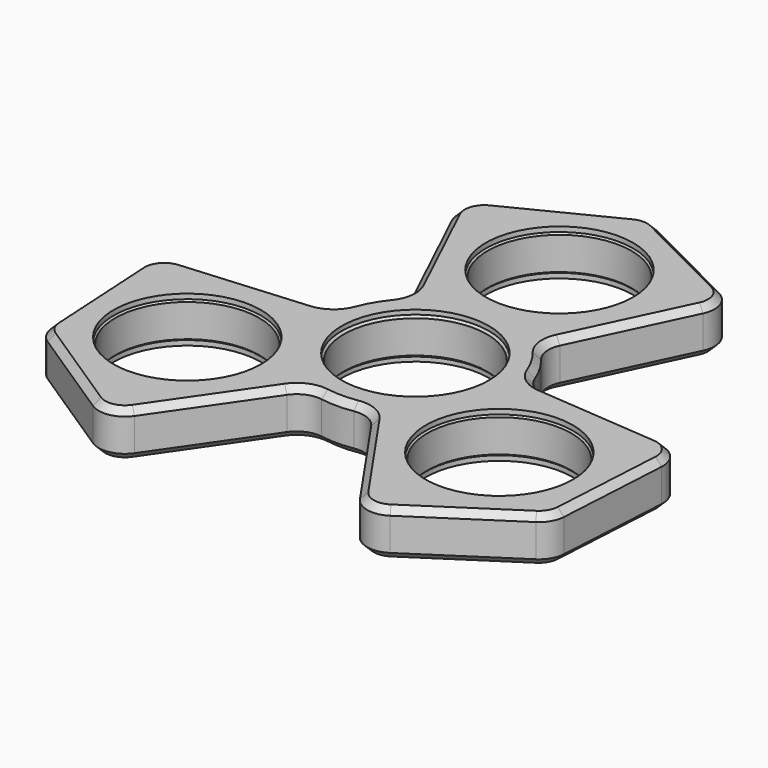
from build123d import *

# Parameters (mm, degrees)
F0_R     = 11
F0_R_2   = 10.925
F1_DEPTH = 7
F2_R     = 4
F3_SIZE  = 1
F4_R     = 11.925
F4_R_2   = 11.25
F4_R_3   = 12
F5_DEPTH = 7


# Not quite as in the source:
# - a feature names something its author has since deleted; it is built from what else it names


with BuildPart() as f1:
    # F0 (on Top) → F1 (new body)
    with BuildSketch(Plane.XY):
        with BuildLine():
            Line((20.8717118949, 34.490134567), (0, 45))
            Line((0, 45), (-20.8717118949, 34.490134567))
            Line((-20.8717118949, 34.490134567), (-9.8614735953, 11.3027137683))
            ThreePointArc((-9.8614735953, 11.3027137683), (0, 15), (9.8614735953, 11.3027137683))
            Line((9.8614735953, 11.3027137683), (20.8717118949, 34.490134567))
        make_face()
        with Locations((0, 27.5248214602)):
            Circle(F0_R, mode=Mode.SUBTRACT)
        with BuildLine():
            ThreePointArc((9.8614735953, 11.3027137683), (0, 15), (-9.8614735953, 11.3027137683))
            ThreePointArc((-9.8614735953, 11.3027137683), (-12.9903810568, 7.5), (-14.7191740527, 2.8889297681))
            ThreePointArc((-14.7191740527, 2.8889297681), (-12.9903810568, -7.5), (-4.8577004574, -14.1916435365))
            ThreePointArc((-4.8577004574, -14.1916435365), (0, -15), (4.8577004574, -14.1916435365))
            ThreePointArc((4.8577004574, -14.1916435365), (12.2038007781, -8.7216538896), (15, 0))
            ThreePointArc((15, 0), (14.9296284413, 1.4512734423), (14.7191740527, 2.8889297681))
            ThreePointArc((14.7191740527, 2.8889297681), (12.9903810568, 7.5), (9.8614735953, 11.3027137683))
        make_face()
        Circle(F0_R_2, mode=Mode.SUBTRACT)
        with BuildLine():
            ThreePointArc((-4.8577004574, -14.1916435365), (-12.9903810568, -7.5), (-14.7191740527, 2.8889297681))
            Line((-14.7191740527, 2.8889297681), (-40.3051886624, 0.8303654379))
            Line((-40.3051886624, 0.8303654379), (-38.9711431703, -22.5))
            Line((-38.9711431703, -22.5), (-19.4334767676, -35.3205000049))
            Line((-19.4334767676, -35.3205000049), (-4.8577004574, -14.1916435365))
        make_face()
        with Locations((-23.8371946192, -13.7624107301)):
            Circle(F0_R, mode=Mode.SUBTRACT)
        with BuildLine():
            Line((40.3051886624, 0.8303654379), (14.7191740527, 2.8889297681))
            ThreePointArc((14.7191740527, 2.8889297681), (14.9296284413, 1.4512734423), (15, 0))
            ThreePointArc((15, 0), (12.2038007781, -8.7216538896), (4.8577004574, -14.1916435365))
            Line((4.8577004574, -14.1916435365), (19.4334767676, -35.3205000049))
            Line((19.4334767676, -35.3205000049), (38.9711431703, -22.5))
            Line((38.9711431703, -22.5), (40.3051886624, 0.8303654379))
        make_face()
        with Locations((23.8371946192, -13.7624107301)):
            Circle(F0_R, mode=Mode.SUBTRACT)
    extrude(amount=F1_DEPTH)

    # F2
    f2_edges = [f1.edges().sort_by_distance(p)[0] for p in [
        (9.861474, 11.302714, 3.5),
        (-9.861474, 11.302714, 3.5),
        (14.719174, 2.88893, 3.5),
        (4.8577, -14.191644, 3.5),
        (-4.8577, -14.191644, 3.5),
        (-14.719174, 2.88893, 3.5),
        (20.871712, 34.490135, 3.5),
        (0, 45, 3.5),
        (-20.871712, 34.490135, 3.5),
        (19.433477, -35.3205, 3.5),
        (38.971143, -22.5, 3.5),
        (40.305189, 0.830365, 3.5),
        (-19.433477, -35.3205, 3.5),
        (-38.971143, -22.5, 3.5),
        (-40.305189, 0.830365, 3.5),
    ]]
    fillet(f2_edges, radius=F2_R)

    # F3
    f3_edges = [f1.edges().sort_by_distance(p)[0] for p in [
        (-15.121499, 22.38026, 7),
        (-15.121499, 22.38026, 0),
        (-39.584098, -11.780379, 7),
        (-29.994156, -28.390645, 7),
        (15.121499, 22.38026, 7),
        (10.691316, 11.594325, 7),
        (19.36544, 33.973357, 7),
        (12.990381, 7.5, 7),
        (9.589942, 40.171024, 7),
        (15.386638, 3.461789, 7),
        (0, 44.521503, 7),
        (26.942623, 1.905472, 7),
        (-9.589942, 40.171024, 7),
        (39.10451, -0.215715, 7),
        (-19.36544, 33.973357, 7),
        (39.584098, -11.780379, 7),
        (38.556753, -22.260751, 7),
        (-10.691316, 11.594325, 7),
        (29.994156, -28.390645, 7),
        (-12.990381, 7.5, 7),
        (19.73907, -33.757641, 7),
        (-15.386638, 3.461789, 7),
        (11.821124, -24.285733, 7),
        (-26.942623, 1.905472, 7),
        (4.695322, -15.056114, 7),
        (-39.10451, -0.215715, 7),
        (0, -15, 7),
        (-4.695322, -15.056114, 7),
        (-38.556753, -22.260751, 7),
        (-11.821124, -24.285733, 7),
        (-19.73907, -33.757641, 7),
        (-11, 27.524821, 7),
        (-10.925, 0, 7),
        (-34.837195, -13.762411, 7),
        (12.837195, -13.762411, 7),
        (15.121499, 22.38026, 0),
        (10.691316, 11.594325, 0),
        (19.36544, 33.973357, 0),
        (12.990381, 7.5, 0),
        (9.589942, 40.171024, 0),
        (15.386638, 3.461789, 0),
        (0, 44.521503, 0),
        (26.942623, 1.905472, 0),
        (-9.589942, 40.171024, 0),
        (39.10451, -0.215715, 0),
        (-19.36544, 33.973357, 0),
        (39.584098, -11.780379, 0),
        (38.556753, -22.260751, 0),
        (-10.691316, 11.594325, 0),
        (29.994156, -28.390645, 0),
        (-12.990381, 7.5, 0),
        (19.73907, -33.757641, 0),
        (-15.386638, 3.461789, 0),
        (11.821124, -24.285733, 0),
        (-26.942623, 1.905472, 0),
        (4.695322, -15.056114, 0),
        (-39.10451, -0.215715, 0),
        (0, -15, 0),
        (-39.584098, -11.780379, 0),
        (-4.695322, -15.056114, 0),
        (-38.556753, -22.260751, 0),
        (-11.821124, -24.285733, 0),
        (-29.994156, -28.390645, 0),
        (-19.73907, -33.757641, 0),
        (-11, 27.524821, 0),
        (-10.925, 0, 0),
        (-34.837195, -13.762411, 0),
        (12.837195, -13.762411, 0),
    ]]
    chamfer(f3_edges, length=F3_SIZE)

    # F4 (on face) → F5 (join)
    with BuildSketch(Plane.XY.offset(7)):
        Circle(F4_R)
        Circle(F4_R_2, mode=Mode.SUBTRACT)
        with Locations((0, 27.5248214602)):
            Circle(F4_R_3)
        with Locations((0, 27.5248214602)):
            Circle(F4_R_2, mode=Mode.SUBTRACT)
        with Locations((-23.8371946192, -13.7624107301)):
            Circle(F4_R_3)
        with Locations((-23.8371946192, -13.7624107301)):
            Circle(F4_R_2, mode=Mode.SUBTRACT)
        with Locations((23.8371946192, -13.7624107301)):
            Circle(F4_R_3)
        with Locations((23.8371946192, -13.7624107301)):
            Circle(F4_R_2, mode=Mode.SUBTRACT)
    extrude(amount=-F5_DEPTH)


solid = f1.part
